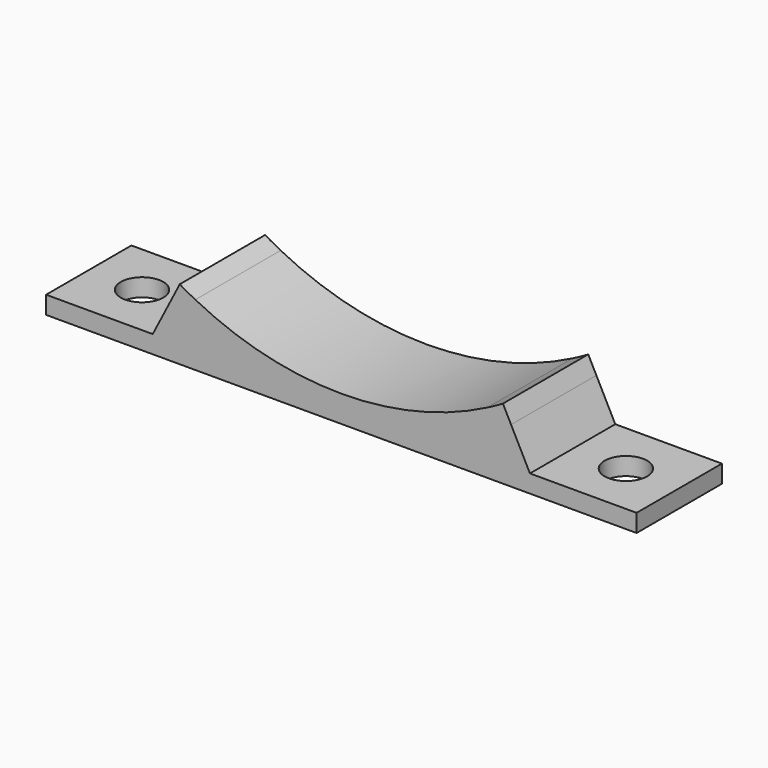
from build123d import *

# Parameters (mm, degrees)
F1_DEPTH = 9.525
F2_R     = 1.89865
F3_DEPTH = 1.5885
F5_DEPTH = 9.525


with BuildPart() as f1:
    # F0 (on Front) → F1 (new body)
    with BuildSketch(Plane.XZ):
        with BuildLine():
            ThreePointArc((13.0392482051, -25.4265339999), (0, -28.575), (-13.0392482051, -25.4265339999))
            Line((-13.0392482051, -25.4265339999), (-13.7636508831, -26.8391192221))
            ThreePointArc((-13.7636508831, -26.8391192221), (0, -30.1625), (13.7636508831, -26.8391192221))
            Line((13.7636508831, -26.8391192221), (13.0392482051, -25.4265339999))
        make_face()
        with BuildLine():
            Line((15.157159657, -26.0775174697), (14.4316955802, -24.66286252))
            ThreePointArc((14.4316955802, -24.66286252), (13.7407782402, -25.0543736372), (13.0392482051, -25.4265339999))
            Line((13.0392482051, -25.4265339999), (13.7636508831, -26.8391192221))
            ThreePointArc((13.7636508831, -26.8391192221), (14.4654184136, -26.4674909345), (15.157159657, -26.0775174697))
        make_face()
        with BuildLine():
            Line((16.844971211, -29.36875), (15.157159657, -26.0775174697))
            ThreePointArc((15.157159657, -26.0775174697), (14.4654184136, -26.4674909345), (13.7636508831, -26.8391192221))
            Line((13.7636508831, -26.8391192221), (15.875, -30.95625))
            Line((15.875, -30.95625), (26.369971211, -30.95625))
            Line((26.369971211, -30.95625), (26.369971211, -29.36875))
            Line((26.369971211, -29.36875), (16.844971211, -29.36875))
        make_face()
        with BuildLine():
            ThreePointArc((-13.0392482051, -25.4265339999), (-13.7407782402, -25.0543736372), (-14.4316955802, -24.66286252))
            Line((-14.4316955802, -24.66286252), (-15.157159657, -26.0775174697))
            ThreePointArc((-15.157159657, -26.0775174697), (-14.4654184136, -26.4674909345), (-13.7636508831, -26.8391192221))
            Line((-13.7636508831, -26.8391192221), (-13.0392482051, -25.4265339999))
        make_face()
        with BuildLine():
            ThreePointArc((-13.7636508831, -26.8391192221), (-14.4654184136, -26.4674909345), (-15.157159657, -26.0775174697))
            Line((-15.157159657, -26.0775174697), (-16.844971211, -29.36875))
            Line((-16.844971211, -29.36875), (-26.369971211, -29.36875))
            Line((-26.369971211, -29.36875), (-26.369971211, -30.95625))
            Line((-26.369971211, -30.95625), (-15.875, -30.95625))
            Line((-15.875, -30.95625), (-13.7636508831, -26.8391192221))
        make_face()
    extrude(amount=F1_DEPTH)

    # F2 (on face) → F3 (cut, through all)
    with BuildSketch(Plane.XY.offset(-29.36875)):
        with Locations((21.607471211, -4.7625)):
            Circle(F2_R)
        with Locations((-21.607471211, -4.7625)):
            Circle(F2_R)
    extrude(amount=-F3_DEPTH, mode=Mode.SUBTRACT)

    # F4 (on face) → F5 (join, through all)
    with BuildSketch(Plane.XZ.offset(9.525)):
        with BuildLine():
            Line((-13.7636508831, -26.8391192221), (-15.875, -30.95625))
            Line((-15.875, -30.95625), (15.875, -30.95625))
            Line((15.875, -30.95625), (13.7636508831, -26.8391192221))
            ThreePointArc((13.7636508831, -26.8391192221), (0, -30.1625), (-13.7636508831, -26.8391192221))
        make_face()
    extrude(amount=-F5_DEPTH)


solid = f1.part
